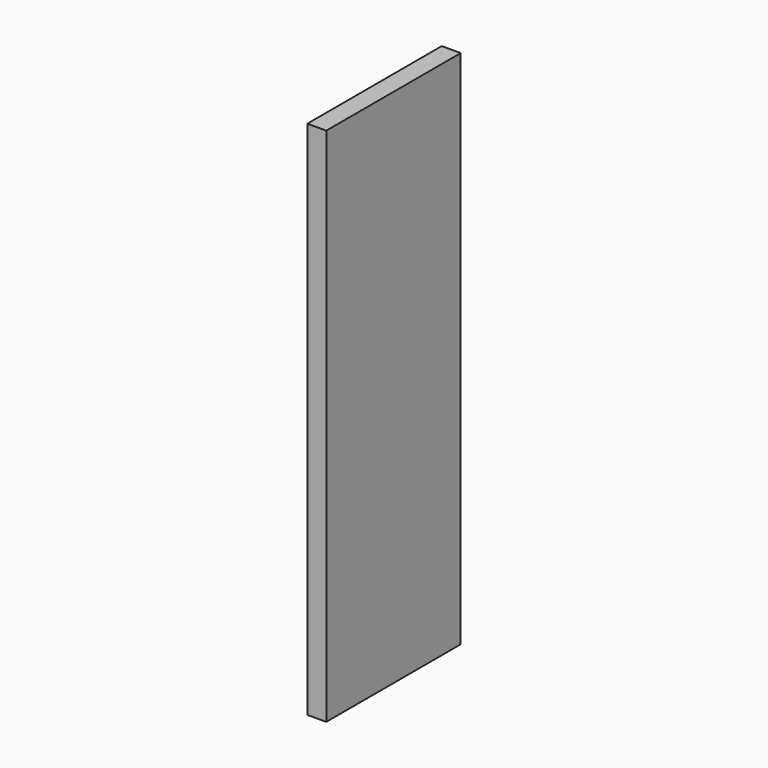
from build123d import *

# Parameters (mm, degrees)
F2_W     = 2.255320549
F2_H     = 6.9872438908
F3_DEPTH = 0.254


# Not quite as in the source:
# - the program builds the solid bodies; features that only make, move or delete a surface that nothing else refers to are left out


with BuildPart() as f3:
    # F2 (on Right) → F3 (new body)
    with BuildSketch(Plane.YZ):
        with Locations((-323.8519430161, 294.0221875906)):
            Rectangle(F2_W, F2_H)
    extrude(amount=F3_DEPTH)


solid = f3.part
